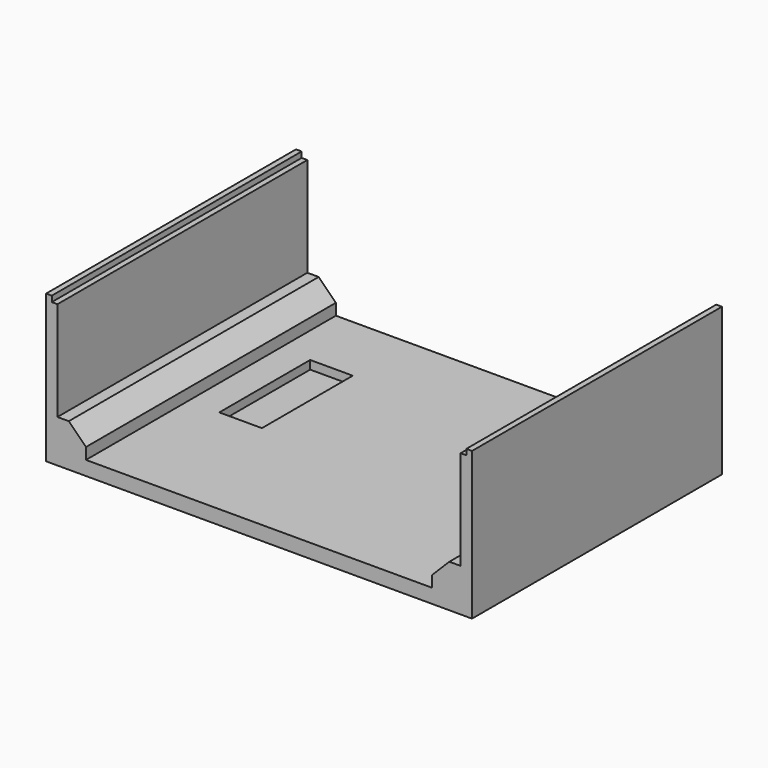
from build123d import *

# Parameters (mm, degrees)
F1_DEPTH = 110
F2_W     = 15
F2_H     = 40
F3_DEPTH = 3


# Not quite as in the source:
# - a feature names something its author has since deleted; it is built from what else it names


with BuildPart() as f1:
    # F0 (on Front) → F1 (new body)
    with BuildSketch(Plane.XZ):
        Polygon((0, 5), (0, 0), (75, 0), (75, 52), (73, 52), (73, 50), (71, 50), (71, 15.0446529165), (67, 15.0446529165), (60.9553470835, 9), (60.9553470835, 5), align=None)
    extrude(amount=F1_DEPTH)

    # F2 (on face) → F3 (cut)
    with BuildSketch(Plane.XY.offset(5)):
        with Locations((42.5, -45)):
            Rectangle(F2_W, F2_H)
    extrude(amount=-F3_DEPTH, mode=Mode.SUBTRACT)

    # F4: F1 across plane


with BuildPart() as f1_1:
    add(f1.part)
    add(f1.part.mirror(Plane.YZ))


solid = f1_1.part
